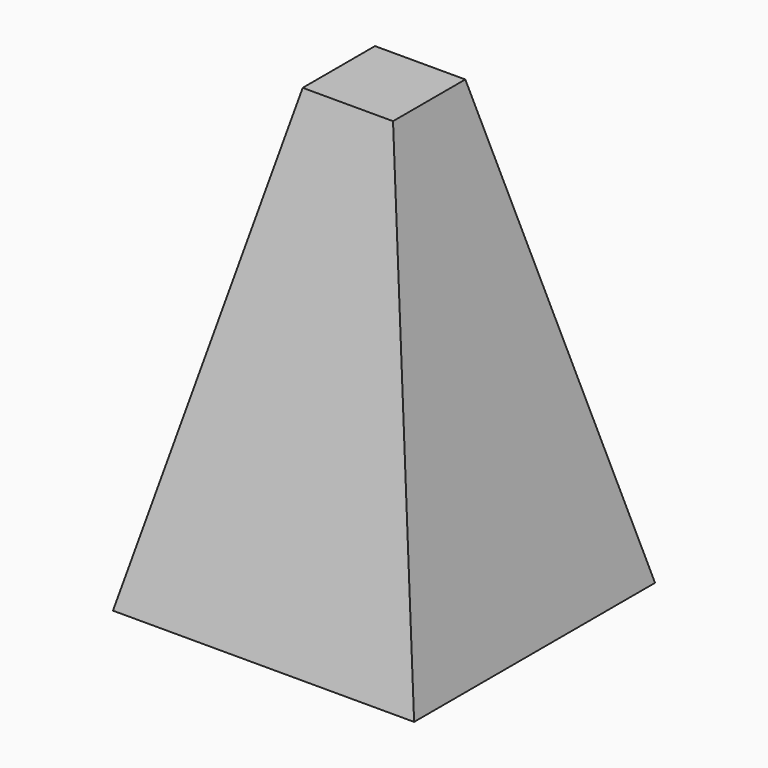
from build123d import *

# Parameters (mm, degrees)
F1_DEPTH = 25
F2_SIZE2 = 74.99999
F2_SIZE  = 17.49999


# Not quite as in the source:
# - a fillet or chamfer is up to 0.001 mm smaller than in the source, because OpenCascade refuses the exact size


with BuildPart() as f1:
    # F0 (on Front) → F1 (new body, symmetric)
    with BuildSketch(Plane.XZ):
        Polygon((25, -29.9881670944), (7.5, 45.0118329056), (-7.5, 45.0118329056), (-25, -29.9881670944), align=None)
    extrude(amount=F1_DEPTH, both=True)

    # F2 (size 17.5 and 75 in the source; OpenCascade refuses exactly that, so slightly less here)
    f2_edges = [f1.edges().sort_by_distance(p)[0] for p in [
        (0, 25, 45.011833),
        (0, -25, 45.011833),
    ]]
    f2_side = f1.faces().sort_by_distance((0, 0, 45.011833))[0]
    chamfer(f2_edges, length=F2_SIZE, length2=F2_SIZE2, reference=f2_side)


solid = f1.part
